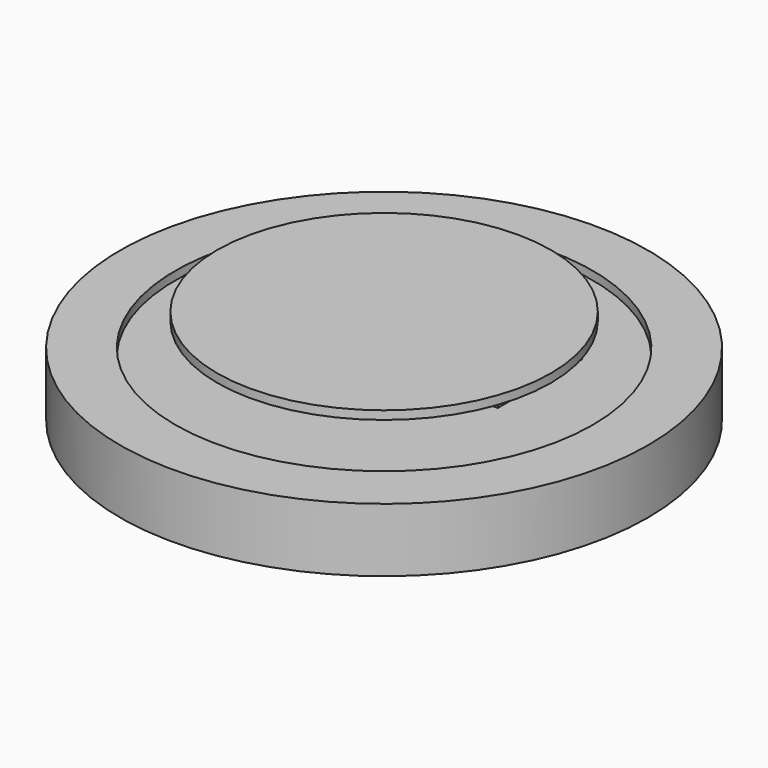
from build123d import *

# Parameters (mm, degrees)
F0_W      = 170.18
F0_H      = 170.18
F1_DEPTH  = 5
F2_W      = 86.7
F2_H      = 49.7
F3_DEPTH  = 37
F6_START  = 11
F5_R      = 118.3354320223
F6_DEPTH  = 3.8
F4_R      = 124.3354320223
F4_R_2    = 120.3354320223
F8_DEPTH  = 26
F9_R      = 124.3354320223
F9_R_2    = 98.3354320223
F10_DEPTH = 4
F12_START = 4
F11_R     = 78.6222719846
F12_DEPTH = 4


# Not quite as in the source:
# - the program builds the solid bodies; features that only make, move or delete a surface that nothing else refers to are left out


with BuildPart() as f1:
    # F0 (on Top) → F1 (new body)
    with BuildSketch(Plane.XY):
        with Locations((85.09, -85.09)):
            Rectangle(F0_W, F0_H)
    extrude(amount=F1_DEPTH)

    # F2 (on face) → F3 (join)
    with BuildSketch(Plane(origin=(0, 0, 0), x_dir=(1, 0, 0), z_dir=(0, 0, -1))):
        with Locations((92.13, 56.25)):
            Rectangle(F2_W, F2_H)
    extrude(amount=-F3_DEPTH)

    # F5 (on face) → F6 (join)
    with BuildSketch(Plane.XY.offset(5).offset(F6_START)):
        with Locations((85.09, -85.09)):
            Circle(F5_R)
    extrude(amount=F6_DEPTH)


with BuildPart() as f8:
    # F4 (on Top) → F8 (new body)
    with BuildSketch(Plane.XY):
        with Locations((85.09, -85.09)):
            Circle(F4_R)
        with Locations((85.09, -85.09)):
            Circle(F4_R_2, mode=Mode.SUBTRACT)
    extrude(amount=F8_DEPTH)

    # F9 (on face) → F10 (join)
    with BuildSketch(Plane.XY.offset(26)):
        with Locations((85.09, -85.09)):
            Circle(F9_R)
        with Locations((85.09, -85.09)):
            Circle(F9_R_2, mode=Mode.SUBTRACT)
    extrude(amount=F10_DEPTH)


with BuildPart() as f12:
    # F11 (on face) → F12 (new body)
    with BuildSketch(Plane.XY.offset(37).offset(F12_START)):
        with Locations((85.09, -85.09)):
            Circle(F11_R)
    extrude(amount=F12_DEPTH)


solid = Compound([f1.part, f8.part, f12.part])
